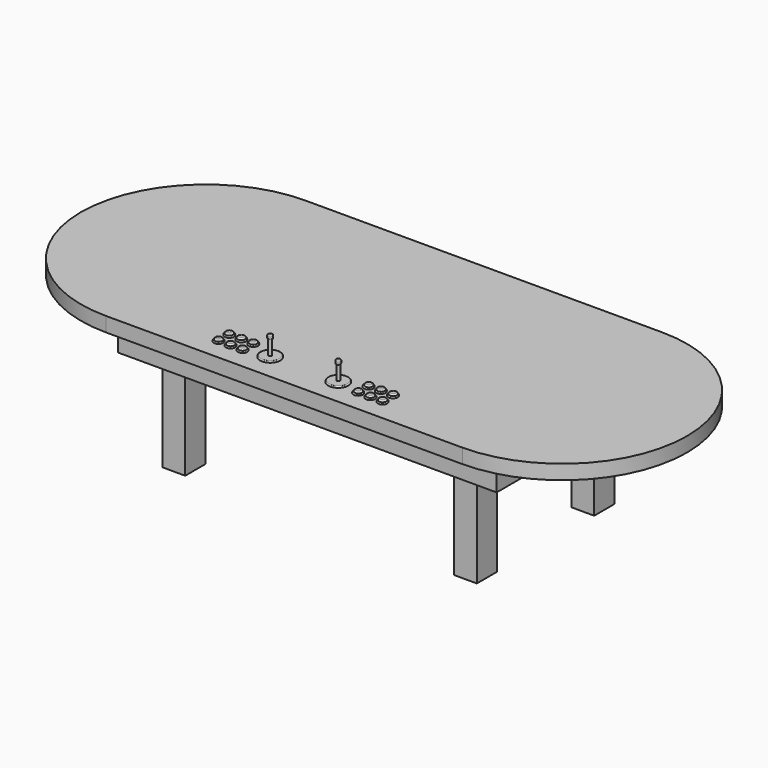
from build123d import *

# Parameters (mm, degrees)
F0_W      = 93.5235582292
F0_H      = 65.5109807849
F1_DEPTH  = 3.81
F2_W      = 99.2795974016
F2_H      = 53.1533658504
F3_DEPTH  = 8.89
F4_W      = 5.9323385358
F4_H      = 6.6234655678
F5_DEPTH  = 25.4
F6_R      = 1.2294027509
F6_R_2    = 2.6396421085
F7_DEPTH  = 0.381
F8_R      = 0.9793123783
F9_DEPTH  = 0.381
F10_R     = 0.254
F11_R     = 0.38099
F12_R     = 0.4115244645
F13_DEPTH = 3.81
F14_R     = 0.6161358957
F15_DEPTH = 1.016


# Not quite as in the source:
# - a fillet or chamfer that OpenCascade refuses, or shapes differently, is made with other operations: its cross-section is extruded or revolved along the edge and cut away or added
# - a fillet or chamfer is up to 0.001 mm smaller than in the source, because OpenCascade refuses the exact size


with BuildPart() as f1:
    # F0 (on Top) → F1 (new body)
    with BuildSketch(Plane.XY):
        with Locations((0.2010185272, -1.7233528197)):
            Rectangle(F0_W, F0_H)
        with BuildLine():
            Line((-46.5607605875, -34.4788432121), (-46.5607605875, 31.0321375728))
            ThreePointArc((-46.5607605875, 31.0321375728), (-79.3162509799, -1.7233528197), (-46.5607605875, -34.4788432121))
        make_face()
        with BuildLine():
            ThreePointArc((46.9627976418, -34.4788432121), (79.7182880342, -1.7233528197), (46.9627976418, 31.0321375728))
            Line((46.9627976418, 31.0321375728), (46.9627976418, -34.4788432121))
        make_face()
    extrude(amount=F1_DEPTH)

    # F2 (on face) → F3 (join)
    with BuildSketch(Plane(origin=(0, 0, 0), x_dir=(1, 0, 0), z_dir=(0, 0, -1))):
        Rectangle(F2_W, F2_H)
    extrude(amount=F3_DEPTH)

    # F4 (on face) → F5 (join)
    with BuildSketch(Plane(origin=(0, 0, -8.89), x_dir=(1, 0, 0), z_dir=(0, 0, -1))):
        with Locations((-38.2571481168, 19.2429218441)):
            Rectangle(F4_W, F4_H)
        with Locations((38.2571481168, 19.2429218441)):
            Rectangle(F4_W, F4_H)
        with Locations((38.2571481168, -19.2429218441)):
            Rectangle(F4_W, F4_H)
        with Locations((-38.2571481168, -19.2429218441)):
            Rectangle(F4_W, F4_H)
    extrude(amount=F5_DEPTH)

    # F6 (on face) → F7 (join)
    with BuildSketch(Plane.XY.offset(3.81)):
        with Locations((-15.1624232531, -28.8937985897)):
            Circle(F6_R)
        with Locations((-15.1305962354, -25.4226885736)):
            Circle(F6_R)
        with Locations((-18.3360408992, -28.8639198989)):
            Circle(F6_R)
        with Locations((-18.3042138815, -25.3928098828)):
            Circle(F6_R)
        with Locations((-21.5096585453, -28.834041208)):
            Circle(F6_R)
        with Locations((-21.4778315276, -25.3629311919)):
            Circle(F6_R)
        with Locations((21.5096585453, -28.834041208)):
            Circle(F6_R)
        with Locations((18.3360408992, -28.8639198989)):
            Circle(F6_R)
        with Locations((21.4778315276, -25.3629311919)):
            Circle(F6_R)
        with Locations((18.3042138815, -25.3928098828)):
            Circle(F6_R)
        with Locations((15.1305962354, -25.4226885736)):
            Circle(F6_R)
        with Locations((15.1624232531, -28.8937985897)):
            Circle(F6_R)
        with Locations((8.924825117, -27.6222340763)):
            Circle(F6_R_2)
        with Locations((-8.924825117, -27.6222340763)):
            Circle(F6_R_2)
    extrude(amount=F7_DEPTH)

    # F8 (on face) → F9 (join)
    with BuildSketch(Plane.XY.offset(4.191)):
        with Locations((21.5035416186, -28.7971198559)):
            Circle(F8_R)
        with Locations((21.4913431555, -25.3196582198)):
            Circle(F8_R)
        with Locations((18.3376446366, -28.8268737495)):
            Circle(F8_R)
        with Locations((18.3254461735, -25.3494121134)):
            Circle(F8_R)
        with Locations((15.1717476547, -28.8566276431)):
            Circle(F8_R)
        with Locations((15.1595491916, -25.379166007)):
            Circle(F8_R)
        with Locations((-15.1717476547, -28.8566276431)):
            Circle(F8_R)
        with Locations((-15.1595491916, -25.379166007)):
            Circle(F8_R)
        with Locations((-18.3254461735, -25.3494121134)):
            Circle(F8_R)
        with Locations((-18.3376446366, -28.8268737495)):
            Circle(F8_R)
        with Locations((-21.5035416186, -28.7971198559)):
            Circle(F8_R)
        with Locations((-21.4913431555, -25.3196582198)):
            Circle(F8_R)
    extrude(amount=F9_DEPTH)

    # F10
    f10_edges = [f1.edges().sort_by_distance(p)[0] for p in [
        (-22.739061, -28.834041, 4.191),
        (-19.565444, -28.86392, 4.191),
        (-16.391826, -28.893799, 4.191),
        (-16.359999, -25.422689, 4.191),
        (-22.707234, -25.362931, 4.191),
        (-19.533617, -25.39281, 4.191),
        (20.280256, -28.834041, 4.191),
        (20.248429, -25.362931, 4.191),
        (13.933021, -28.893799, 4.191),
        (17.074811, -25.39281, 4.191),
        (13.901193, -25.422689, 4.191),
        (-11.564467, -27.622234, 4.191),
        (6.285183, -27.622234, 4.191),
        (17.106638, -28.86392, 4.191),
    ]]
    fillet(f10_edges, radius=F10_R)

    # F11 (radius 0.381 in the source; OpenCascade refuses exactly that, so slightly less here)
    f11_edges = [f1.edges().sort_by_distance(p)[0] for p in [
        (-22.482854, -28.79712, 4.572),
        (-22.470656, -25.319658, 4.572),
        (-19.304759, -25.349412, 4.572),
        (-19.316957, -28.826874, 4.572),
        (-16.138862, -25.379166, 4.572),
        (-16.15106, -28.856628, 4.572),
        (14.180237, -25.379166, 4.572),
        (14.192435, -28.856628, 4.572),
        (17.346134, -25.349412, 4.572),
        (17.358332, -28.826874, 4.572),
        (20.524229, -28.79712, 4.572),
        (20.512031, -25.319658, 4.572),
    ]]
    fillet(f11_edges, radius=F11_R)

    # F12 (on face) → F13 (join)
    with BuildSketch(Plane.XY.offset(4.191)):
        with Locations((-8.924825117, -27.6222340763)):
            Circle(F12_R)
        with Locations((8.924825117, -27.6222340763)):
            Circle(F12_R)
    extrude(amount=F13_DEPTH)

    # F14 (on face) → F15 (join)
    with BuildSketch(Plane.XY.offset(8.001)):
        with Locations((-8.924825117, -27.6222340763)):
            Circle(F14_R)
        with Locations((8.924825117, -27.6222340763)):
            Circle(F14_R)
    extrude(amount=F15_DEPTH)

    # F16: fillet of radius 0.254 on 4 edges, made by hand

    # F16_s1 → F16_t2 (revolve, cut)
    with BuildSketch(Plane.XZ.offset(27.6222340763)):
        with BuildLine():
            ThreePointArc((-8.3086892213, 8.2501521007), (-8.3663977334, 8.0889514438), (-8.5133006525, 8.001))
            Line((-8.5133006525, 8.001), (-8.5123128812, 7.996016958))
            ThreePointArc((-8.5123128812, 7.996016958), (-8.4109949369, 7.99592), (-8.3086892213, 7.99592))
            Line((-8.3086892213, 7.99592), (-8.3036092213, 8.001))
            Line((-8.3036092213, 8.001), (-8.3036092213, 8.2501521007))
            Line((-8.3036092213, 8.2501521007), (-8.3086892213, 8.2501521007))
        make_face()
    revolve(axis=Axis((-8.924825117, -27.6222340763, 8.001), (0, 0, 1)), mode=Mode.SUBTRACT)

    # F16_s3 → F16_t4 (revolve, cut)
    with BuildSketch(Plane.XZ.offset(27.6222340763)):
        with BuildLine():
            ThreePointArc((-8.3086892213, 8.763), (-8.3830840989, 8.9426051224), (-8.5626892213, 9.017))
            Line((-8.5626892213, 9.017), (-8.5626892213, 9.02208))
            Line((-8.5626892213, 9.02208), (-8.3036092213, 9.02208))
            Line((-8.3036092213, 9.02208), (-8.3036092213, 8.763))
            Line((-8.3036092213, 8.763), (-8.3086892213, 8.763))
        make_face()
    revolve(axis=Axis((-8.924825117, -27.6222340763, 9.017), (0, 0, 1)), mode=Mode.SUBTRACT)

    # F16_s5 → F16_t6 (revolve, cut)
    with BuildSketch(Plane.XZ.offset(27.6222340763)):
        with BuildLine():
            ThreePointArc((9.5409610127, 8.763), (9.4665661351, 8.9426051224), (9.2869610127, 9.017))
            Line((9.2869610127, 9.017), (9.2869610127, 9.02208))
            Line((9.2869610127, 9.02208), (9.5460410127, 9.02208))
            Line((9.5460410127, 9.02208), (9.5460410127, 8.763))
            Line((9.5460410127, 8.763), (9.5409610127, 8.763))
        make_face()
    revolve(axis=Axis((8.924825117, -27.6222340763, 9.017), (0, 0, 1)), mode=Mode.SUBTRACT)

    # F16_s7 → F16_t8 (revolve, cut)
    with BuildSketch(Plane.XZ.offset(27.6222340763)):
        with BuildLine():
            ThreePointArc((9.3363495815, 8.001), (9.4832525006, 8.0889514438), (9.5409610127, 8.2501521007))
            Line((9.5409610127, 8.2501521007), (9.5460410127, 8.2501521007))
            Line((9.5460410127, 8.2501521007), (9.5460410127, 8.001))
            Line((9.5460410127, 8.001), (9.5409610127, 7.99592))
            ThreePointArc((9.5409610127, 7.99592), (9.4386552971, 7.99592), (9.3373373528, 7.996016958))
            Line((9.3373373528, 7.996016958), (9.3363495815, 8.001))
        make_face()
    revolve(axis=Axis((8.924825117, -27.6222340763, 8.001), (0, 0, 1)), mode=Mode.SUBTRACT)


solid = f1.part
